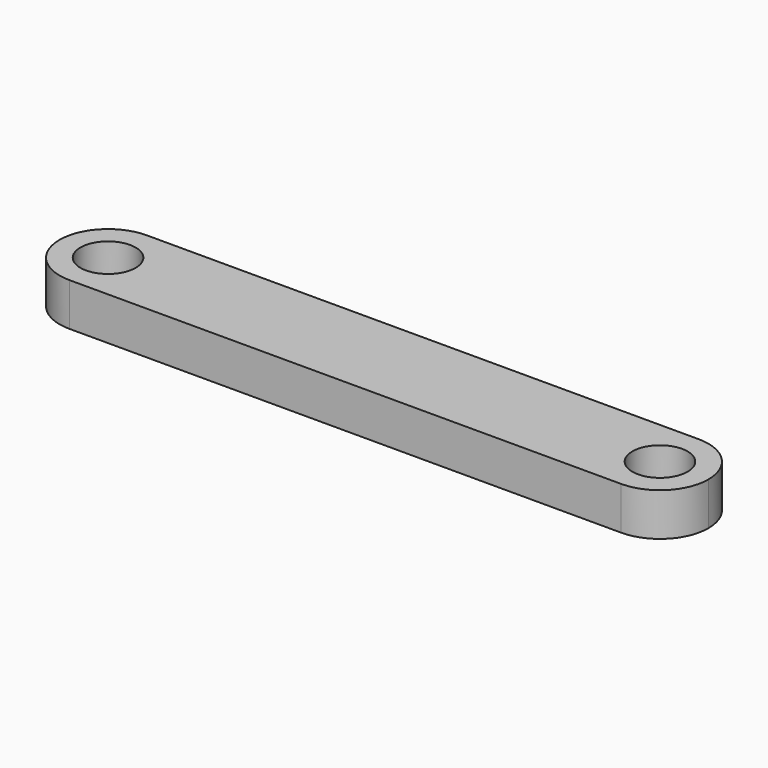
from build123d import *

# Parameters (mm, degrees)
F0_R     = 5.715
F1_DEPTH = 8.89


# Not quite as in the source:
# - the program builds the solid bodies; features that only make, move or delete a surface that nothing else refers to are left out


with BuildPart() as f1:
    # F0 (on Top) → F1 (new body)
    with BuildSketch(Plane.XY):
        with BuildLine():
            ThreePointArc((-87.9825091655, 10.033), (-80.8881068298, 7.0944023356), (-77.9495091655, 0))
            ThreePointArc((-77.9495091655, 0), (-80.8881068298, -7.0944023356), (-87.9825091655, -10.033))
            Line((-87.9825091655, -10.033), (26.3174908345, -10.033))
            ThreePointArc((26.3174908345, -10.033), (16.2844908345, 0), (26.3174908345, 10.033))
            Line((26.3174908345, 10.033), (-87.9825091655, 10.033))
        make_face()
        with BuildLine():
            ThreePointArc((-87.9825091655, -10.033), (-80.8881068298, -7.0944023356), (-77.9495091655, 0))
            ThreePointArc((-77.9495091655, 0), (-80.8881068298, 7.0944023356), (-87.9825091655, 10.033))
            ThreePointArc((-87.9825091655, 10.033), (-98.0155091655, 0), (-87.9825091655, -10.033))
        make_face()
        with Locations((-87.9825091655, 0)):
            Circle(F0_R, mode=Mode.SUBTRACT)
        with BuildLine():
            ThreePointArc((36.3504908345, 0), (33.4118931702, 7.0944023356), (26.3174908345, 10.033))
            ThreePointArc((26.3174908345, 10.033), (16.2844908345, 0), (26.3174908345, -10.033))
            ThreePointArc((26.3174908345, -10.033), (33.4118931702, -7.0944023356), (36.3504908345, 0))
        make_face()
        with Locations((26.3174908345, 0)):
            Circle(F0_R, mode=Mode.SUBTRACT)
    extrude(amount=F1_DEPTH)


solid = f1.part
